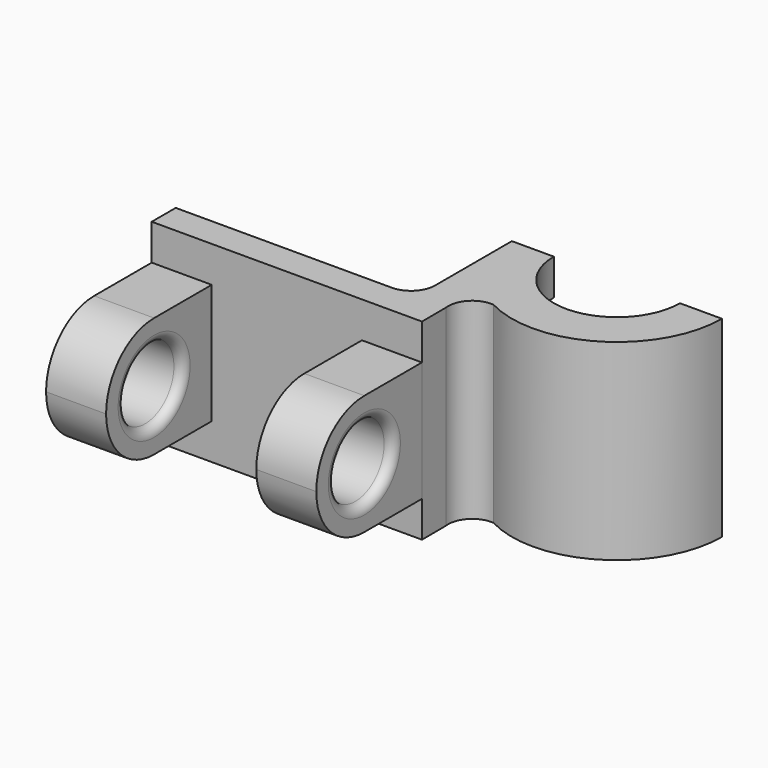
from build123d import *

# Parameters (mm, degrees)
F1_DEPTH = 16
F2_DEPTH = 4
F3_DEPTH = 10
F4_W     = 10
F4_H     = 20
F5_DEPTH = 22
F6_R     = 6
F7_DEPTH = 75.0009999306
F8_R     = 1.5


# Not quite as in the source:
# - ends of sketch curves that miss each other by under 0.0002 mm in the source are joined


with BuildPart() as f1:
    # F0 (on Top) → F1 (new body, symmetric)
    with BuildSketch(Plane.XY):
        Polygon((14.1706688348, 5), (5.1815587922, 5), (-30.8302634659, 5), (-30.8302634659, 0), (14.1933665337, 0), align=None)
        with BuildLine():
            ThreePointArc((9.1762328499, 9.2063472144), (8.0820233117, 6.2454935885), (5.1815587922, 5))
            Line((5.1815587922, 5), (14.1706688348, 5))
            ThreePointArc((14.1706688348, 5), (15.2379483, 8.3057115079), (18.4888007758, 9.5299550339))
            ThreePointArc((18.4888007758, 9.5299550339), (35.6997870029, 10.0097302467), (44.1697364647, 25))
            Line((44.1697364647, 25), (39.1697364647, 25))
            ThreePointArc((39.1697364647, 25), (26.6697364647, 12.5), (14.1697364647, 25))
            Line((14.1697364647, 25), (9.169736973, 25))
            Line((9.169736973, 25), (9.1697442854, 24.9834553538))
            Line((9.1697442854, 24.9834553538), (9.1762328499, 9.2063472144))
        make_face()
        with BuildLine():
            Line((14.1706688348, 25), (14.1697364647, 25))
            ThreePointArc((14.1697364647, 25), (26.6697364647, 12.5), (39.1697364647, 25))
            Line((39.1697364647, 25), (37.1697364647, 25))
            ThreePointArc((37.1697364647, 25), (26.6697364647, 14.5), (16.1697364647, 25))
            Line((16.1697364647, 25), (14.1706688348, 25))
        make_face()
    extrude(amount=F1_DEPTH, both=True)

    # F0 (on Top) → F2 (join, symmetric)
    with BuildSketch(Plane.XY):
        with BuildLine():
            Line((-30.8302634659, 5), (5.1815587922, 5))
            ThreePointArc((5.1815587922, 5), (8.0820233117, 6.2454935885), (9.1762328499, 9.2063472144))
            Line((9.1762328499, 9.2063472144), (9.1697442854, 24.9834553538))
            Line((9.1697442854, 24.9834553538), (9.1697374812, 25.0000000002))
            Line((9.1697374812, 25.0000000002), (9.168883179, 25))
            Line((9.168883179, 25), (-30.8302634659, 5))
        make_face()
    extrude(amount=F2_DEPTH, both=True)

    # F0 (on Top) → F3 (cut, symmetric)
    with BuildSketch(Plane.XY):
        with BuildLine():
            Line((14.1706688348, 25), (14.1697364647, 25))
            ThreePointArc((14.1697364647, 25), (26.6697364647, 12.5), (39.1697364647, 25))
            Line((39.1697364647, 25), (37.1697364647, 25))
            ThreePointArc((37.1697364647, 25), (26.6697364647, 14.5), (16.1697364647, 25))
            Line((16.1697364647, 25), (14.1706688348, 25))
        make_face()
    extrude(amount=F3_DEPTH, both=True, mode=Mode.SUBTRACT)

    # F4 (on face) → F5 (join)
    with BuildSketch(Plane.XZ):
        with Locations((9.1933665337, 0)):
            Rectangle(F4_W, F4_H)
        Polygon((-20.8302634659, 10), (-30.8302634659, 10), (-30.8302634659, 0), (-30.8302634659, -10), (-20.8302634659, -10), align=None)
    extrude(amount=F5_DEPTH)

    # F6 (on face) → F7 (cut, through all)
    with BuildSketch(Plane(origin=(-30.8302634659, 0, 0), x_dir=(0, -1, 0), z_dir=(-1, 0, 0))):
        with BuildLine():
            Line((22, 10), (12, 10))
            ThreePointArc((12, 10), (19.0710677836, 7.0710678402), (22, 8.01e-08))
            Line((22, 8.01e-08), (22, 10))
        make_face()
        with BuildLine():
            Line((22, -10), (22, 8.01e-08))
            ThreePointArc((22, 8.01e-08), (19.0710678402, -7.0710677836), (12, -10))
            Line((12, -10), (22, -10))
        make_face()
        with Locations((12, 0)):
            Circle(F6_R)
    extrude(amount=-F7_DEPTH, mode=Mode.SUBTRACT)

    # F8
    f8_edges = [f1.edges().sort_by_distance(p)[0] for p in [
        (-30.830263, -6, 0),
        (-20.830263, -6, 0),
        (14.193367, -6, 0),
        (4.193367, -6, 0),
    ]]
    fillet(f8_edges, radius=F8_R)


solid = f1.part
